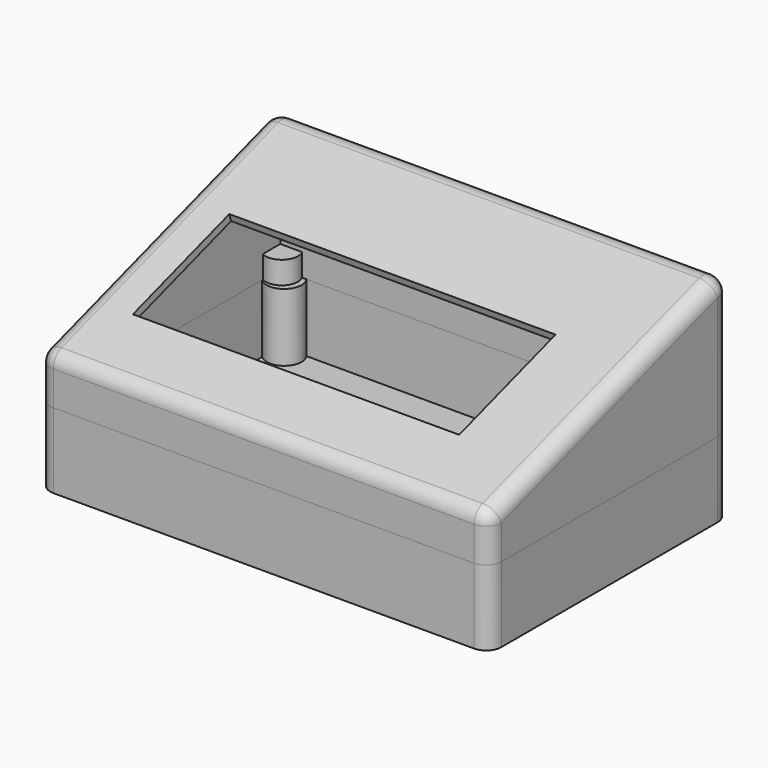
from build123d import *

# Parameters (mm, degrees)
F0_W      = 150
F0_H      = 100
F1_DEPTH  = 25
F2_R      = 3.2981256226
F2_R_2    = 3.2107397339
F2_R_3    = 2.9330141842
F2_R_4    = 4.4377369933
F3_DEPTH  = 25.001
F4_T      = -2.5
F6_DEPTH  = 150
F7_R      = 2.8661980647
F7_R_2    = 2.890017818
F7_R_3    = 3.1801309688
F7_R_4    = 2.9402334405
F8_DEPTH  = 5
F9_T      = 2.5
F10_W     = 108.5215471685
F10_H     = 42.1287603676
F11_DEPTH = 69.0646432345
F12_R     = 5
F13_R     = 5


# Not quite as in the source:
# - a shell that OpenCascade refuses in one call is made with other operations: the cavity is built on its own and cut out


with BuildPart() as f1:
    # F0 (on Top) → F1 (new body)
    with BuildSketch(Plane.XY):
        Rectangle(F0_W, F0_H)
    extrude(amount=F1_DEPTH)

    # F2 (on face) → F3 (cut, through all)
    with BuildSketch(Plane.XY.offset(25)):
        with Locations((-68.5258954763, 44.1285409033)):
            Circle(F2_R)
        with Locations((-69.8590800166, -45.1950915158)):
            Circle(F2_R_2)
        with Locations((68.2592540979, -45.4617291689)):
            Circle(F2_R_3)
        with Locations((69.059163332, 42.5287149847)):
            Circle(F2_R_4)
    extrude(amount=-F3_DEPTH, mode=Mode.SUBTRACT)

    # F4
    f4_openings = [f1.faces().sort_by_distance(p)[0] for p in [
        (-0.101934, -0.097469, 25),
    ]]
    offset(amount=F4_T, openings=f4_openings)

    # F13
    f13_edges = [f1.edges().sort_by_distance(p)[0] for p in [
        (-75, -50, 12.5),
        (75, -50, 12.5),
        (75, 50, 12.5),
        (-75, 50, 12.5),
    ]]
    fillet(f13_edges, radius=F13_R)


with BuildPart() as f6:
    # F5 (on face) → F6 (new body, through all)
    with BuildSketch(Plane(origin=(-75, 0, 0), x_dir=(0, -1, 0), z_dir=(-1, 0, 0))):
        Polygon((-50, 72.6446807384), (-50, 25), (50, 25), (50, 40.0270335376), align=None)
    extrude(amount=-F6_DEPTH)

    # F7 (on face) → F8 (cut)
    with BuildSketch(Plane(origin=(0, 0, 25), x_dir=(1, 0, 0), z_dir=(0, 0, -1))):
        with Locations((-70, 45)):
            Circle(F7_R)
        with Locations((-70, -45)):
            Circle(F7_R_2)
        with Locations((70, -45)):
            Circle(F7_R_3)
        with Locations((70, 45)):
            Circle(F7_R_4)
    extrude(amount=-F8_DEPTH, mode=Mode.SUBTRACT)

    # F9: shell of thickness 2.5, made by hand


with BuildPart() as f9_core1:
    # F9_t2: copy of F6
    add(f6.part)

    # the walls: a layer under each face that stays
    f9_faces = [f9_core1.faces().sort_by_distance(p)[0] for p in [
        (0, 0, 56.335857138),
        (0, -50, 32.5135167688),
        (0, 50, 48.8223403692),
        (-75, 0, 48.8223403692),
        (75, 0, 48.8223403692),
        (66.8198690312, 45, 27.5),
        (67.0597665595, -45, 27.5),
        (-72.890017818, 45, 27.5),
        (-72.8661980647, -45, 27.5),
        (70, 45, 30),
        (70, -45, 30),
        (-70, 45, 30),
        (-70, -45, 30),
    ]]
    thicken(f9_faces, amount=-F9_T, mode=Mode.SUBTRACT)

    # F9_s3 → F9_t4 (revolve, cut)
    with BuildSketch(Plane.XZ.offset(-45)):
        Polygon((73.1551309688, 29.975), (75.6801309688, 30), (75.6801309688, 32.5), (73.1801309688, 32.5), align=None)
    revolve(axis=Axis((70, 45, 30), (0, 0, -1)), mode=Mode.SUBTRACT)

    # F9_s5 → F9_t6 (revolve, cut)
    with BuildSketch(Plane.XZ.offset(45)):
        Polygon((72.9152334405, 29.975), (75.4402334405, 30), (75.4402334405, 32.5), (72.9402334405, 32.5), align=None)
    revolve(axis=Axis((70, -45, 30), (0, 0, -1)), mode=Mode.SUBTRACT)

    # F9_s7 → F9_t8 (revolve, cut)
    with BuildSketch(Plane.XZ.offset(-45)):
        Polygon((-67.134982182, 29.975), (-64.609982182, 30), (-64.609982182, 32.5), (-67.109982182, 32.5), align=None)
    revolve(axis=Axis((-70, 45, 30), (0, 0, -1)), mode=Mode.SUBTRACT)

    # F9_s9 → F9_t10 (revolve, cut)
    with BuildSketch(Plane.XZ.offset(45)):
        Polygon((-67.1588019353, 29.975), (-64.6338019353, 30), (-64.6338019353, 32.5), (-67.1338019353, 32.5), align=None)
    revolve(axis=Axis((-70, -45, 30), (0, 0, -1)), mode=Mode.SUBTRACT)


with BuildPart() as f6_1:
    add(f6.part)

    # what is left inside the walls is the cavity
    f9_cavity = [f9_core1.part.solids().sort_by_distance(p)[0] for p in [
        (24.166667, 0.007752, 53.682461),
    ]]
    add(f9_cavity, mode=Mode.SUBTRACT)

    # F10 (on face) → F11 (cut, through all)
    with BuildSketch(Plane(origin=(0, -16.6084409755, 50.9185744551), x_dir=(1, 0, 0), z_dir=(0, -0.3100975221, 0.9507047527))):
        with Locations((-6.1326678842, 8.1372950226)):
            Rectangle(F10_W, F10_H)
    extrude(amount=-F11_DEPTH, mode=Mode.SUBTRACT)

    # F12
    f12_edges = [f6_1.edges().sort_by_distance(p)[0] for p in [
        (0, 50, 72.644681),
        (-75, 0, 56.335857),
        (75, 0, 56.335857),
        (0, -50, 40.027034),
        (-75, -50, 32.513517),
        (75, -50, 32.513517),
        (75, 50, 48.82234),
        (-75, 50, 48.82234),
    ]]
    fillet(f12_edges, radius=F12_R)


solid = Compound([f1.part, f6_1.part])
